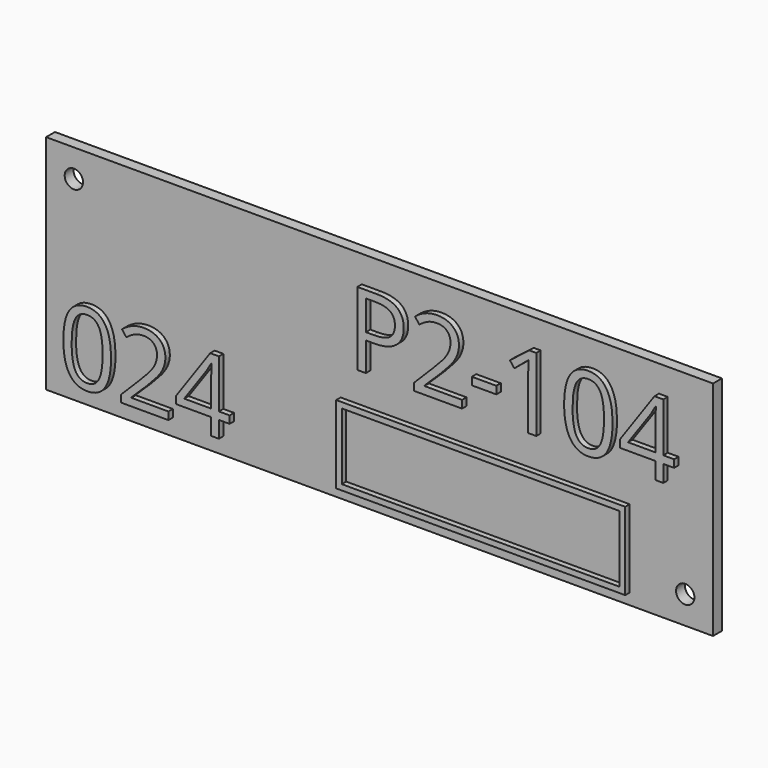
from build123d import *

# Parameters (mm, degrees)
F0_W         = 120
F0_H         = 40
F1_DEPTH     = 2
F3_D         = 3.3
F4_TEXT_SIZE = 18.430525558
F5_DEPTH     = 1
F6_TEXT_SIZE = 18.1818181818
F7_DEPTH     = 1
F8_W         = 52
F8_H         = 14
F8_W_2       = 49.99999962
F8_H_2       = 11.99999962
F9_DEPTH     = 1


# Not quite as in the source:
# - Text() gives the source's letters only with a copy of the font that has no kerning and outlines rounded to 1/6400 em; it was checked with that copy


with BuildPart() as f1:
    # F0 (on Front) → F1 (new body)
    with BuildSketch(Plane.XZ):
        Rectangle(F0_W, F0_H)
    extrude(amount=F1_DEPTH)

    # F3 (through all)
    with Locations(Plane.XZ.offset(2)):
        with Locations((-55, 15), (55, -15)):
            Hole(F3_D / 2)

    # F4 (on face) → F5 (join)
    with BuildSketch(Plane.XZ.offset(2)):
        with Locations((-5, 2)):
            Text('P2-104', F4_TEXT_SIZE, font='Open Sans', text_align=(TextAlign.LEFT, TextAlign.BOTTOM))
    extrude(amount=F5_DEPTH)

    # F6 (on face) → F7 (join)
    with BuildSketch(Plane.XZ.offset(2)):
        with Locations((-57, -17)):
            Text('024', F6_TEXT_SIZE, font='Open Sans', text_align=(TextAlign.LEFT, TextAlign.BOTTOM))
    extrude(amount=F7_DEPTH)

    # F8 (on face) → F9 (join)
    with BuildSketch(Plane.XZ.offset(2)):
        with Locations((19, -11)):
            Rectangle(F8_W, F8_H)
        with Locations((19, -11)):
            Rectangle(F8_W_2, F8_H_2, mode=Mode.SUBTRACT)
    extrude(amount=F9_DEPTH)


solid = f1.part
